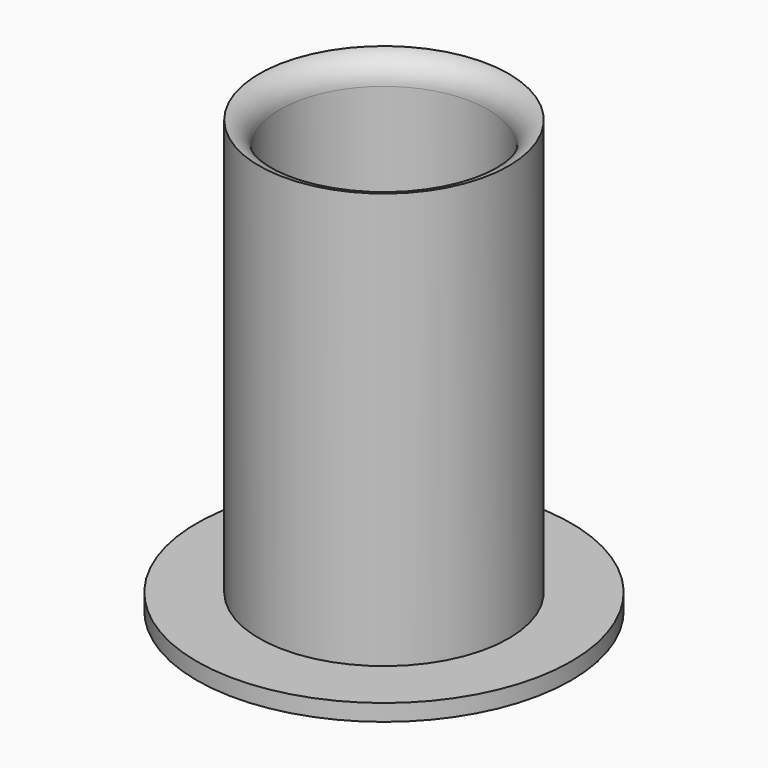
from build123d import *

# Parameters (mm, degrees)
F0_R     = 22.5
F0_R_2   = 12.5
F1_DEPTH = 2
F2_R     = 15
F2_R_2   = 12.5
F3_DEPTH = 50


# Not quite as in the source:
# - a fillet or chamfer that OpenCascade refuses, or shapes differently, is made with other operations: its cross-section is extruded or revolved along the edge and cut away or added


with BuildPart() as f1:
    # F0 (on Top) → F1 (new body)
    with BuildSketch(Plane.XY):
        Circle(F0_R)
        Circle(F0_R_2, mode=Mode.SUBTRACT)
    extrude(amount=F1_DEPTH)

    # F2 (on face) → F3 (join)
    with BuildSketch(Plane.XY.offset(2)):
        Circle(F2_R)
        Circle(F2_R_2, mode=Mode.SUBTRACT)
    extrude(amount=F3_DEPTH)

    # F4: fillet of radius 3 on 2 edges, made by hand

    # F4_s1 → F4_t2 (revolve, cut)
    with BuildSketch(Plane.XZ):
        with BuildLine():
            ThreePointArc((12.5, 3), (13.3786796564, 0.8786796564), (15.5, 0))
            Line((15.5, 0), (12.5, 0))
            Line((12.5, 0), (12.5, 3))
        make_face()
    revolve(axis=Axis((0, 0, 0), (0, 0, 1)), mode=Mode.SUBTRACT)

    # F4_s3 → F4_t4 (revolve, cut)
    with BuildSketch(Plane.XZ):
        with BuildLine():
            ThreePointArc((15, 52), (13.2087121525, 50.9784517816), (12.5, 49.0419601084))
            Line((12.5, 49.0419601084), (12.5, 52))
            Line((12.5, 52), (15, 52))
        make_face()
    revolve(axis=Axis((0, 0, 52), (0, 0, 1)), mode=Mode.SUBTRACT)


solid = f1.part
